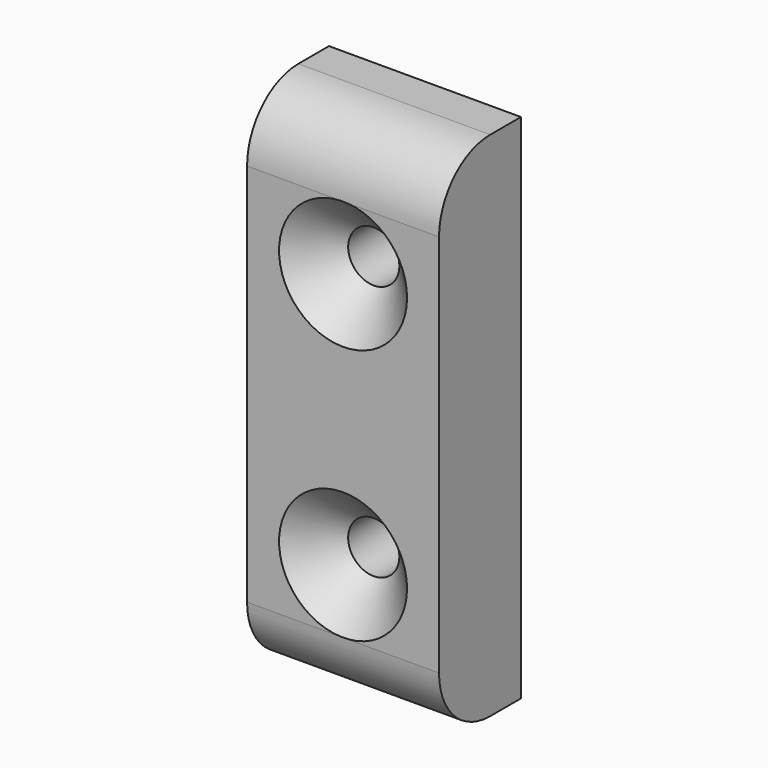
from build123d import *

# Parameters (mm, degrees)
F0_R     = 2
F1_DEPTH = 8
F2_SIZE  = 3
F3_R     = 4.99999


# Not quite as in the source:
# - a fillet or chamfer is up to 0.001 mm smaller than in the source, because OpenCascade refuses the exact size


with BuildPart() as f1:
    # F0 (on Front) → F1 (new body)
    with BuildSketch(Plane.XZ):
        Polygon((0, 20), (0, 0), (0, -20), (15, -20), (15, 0), (15, 20), align=None)
        with Locations((7.5, -10)):
            Circle(F0_R, mode=Mode.SUBTRACT)
        with Locations((7.5, 10)):
            Circle(F0_R, mode=Mode.SUBTRACT)
    extrude(amount=F1_DEPTH)

    # F2
    f2_edges = [f1.edges().sort_by_distance(p)[0] for p in [
        (5.5, -8, 10),
        (5.5, -8, -10),
    ]]
    chamfer(f2_edges, length=F2_SIZE)

    # F3 (radius 5 in the source; OpenCascade refuses exactly that, so slightly less here)
    f3_edges = [f1.edges().sort_by_distance(p)[0] for p in [
        (7.5, -8, 20),
        (7.5, -8, -20),
    ]]
    fillet(f3_edges, radius=F3_R)


solid = f1.part
